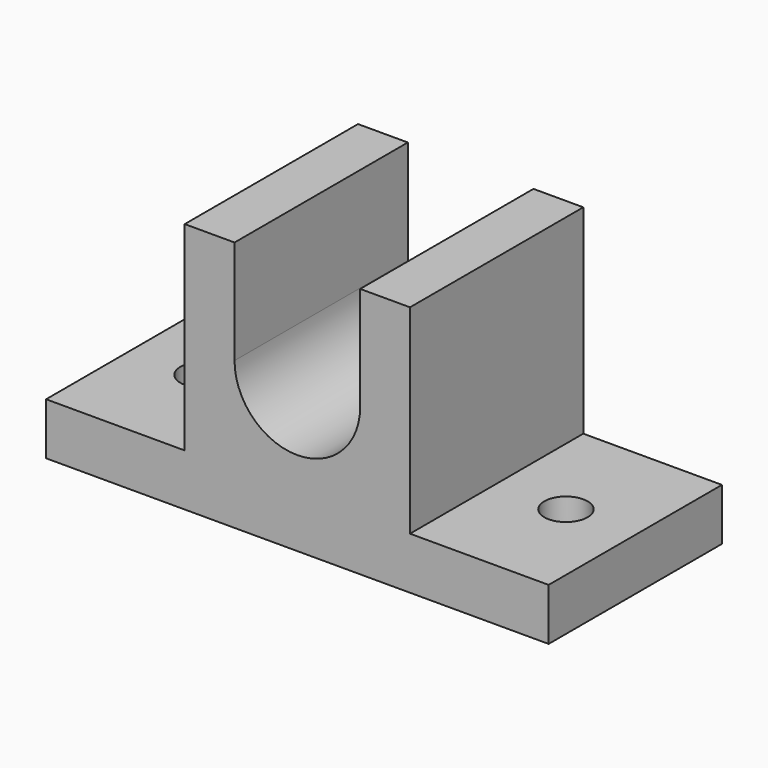
from build123d import *

# Parameters (mm, degrees)
F1_DEPTH = 25
F2_R     = 2.5
F3_DEPTH = 6.001


# Not quite as in the source:
# - a feature names something its author has since deleted; it is built from what else it names


with BuildPart() as f1:
    # F0 (on Front) → F1 (new body)
    with BuildSketch(Plane.XZ):
        with BuildLine():
            ThreePointArc((13, 0), (0, -13), (-13, 0))
            Line((-13, 0), (-13, -11))
            Line((-13, -11), (-29, -11))
            Line((-29, -11), (-29, -17))
            Line((-29, -17), (29, -17))
            Line((29, -17), (29, -11))
            Line((29, -11), (13, -11))
            Line((13, -11), (13, 0))
        make_face()
        with BuildLine():
            Line((-13, 12), (-13, 0))
            ThreePointArc((-13, 0), (0, -13), (13, 0))
            Line((13, 0), (13, 12))
            Line((13, 12), (7.25, 12))
            Line((7.25, 12), (7.25, 0))
            ThreePointArc((7.25, 0), (0, -7.25), (-7.25, 0))
            Line((-7.25, 0), (-7.25, 12))
            Line((-7.25, 12), (-13, 12))
        make_face()
    extrude(amount=F1_DEPTH)

    # F2 (on face) → F3 (cut, through all)
    with BuildSketch(Plane.XY.offset(-11)):
        with Locations((20.9999978542, -12.5)):
            Circle(F2_R)
        with Locations((-20.9999978542, -12.5)):
            Circle(F2_R)
    extrude(amount=-F3_DEPTH, mode=Mode.SUBTRACT)


solid = f1.part
